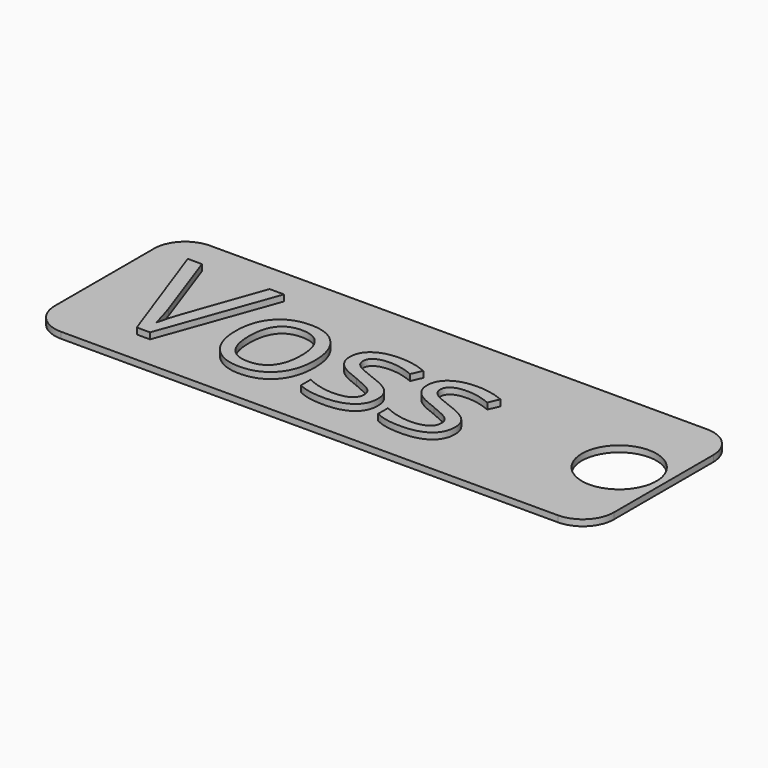
from build123d import *

# Parameters (mm, degrees)
F0_W         = 90
F0_H         = 30
F1_DEPTH     = 1
F2_R         = 5
F3_TEXT_SIZE = 26.041668995
F4_DEPTH     = 1
F6_D         = 12
F6_DEPTH     = 15.5
F6_TIP       = 3.6051637142


# Not quite as in the source:
# - Text() gives the source's letters only with a copy of the font that has no kerning and outlines rounded to 1/6400 em; it was checked with that copy


with BuildPart() as f1:
    # F0 (on Top) → F1 (new body)
    with BuildSketch(Plane.XY):
        Rectangle(F0_W, F0_H)
    extrude(amount=F1_DEPTH)

    # F2
    f2_edges = [f1.edges().sort_by_distance(p)[0] for p in [
        (-45, -15, 0.5),
        (45, -15, 0.5),
        (45, 15, 0.5),
        (-45, 15, 0.5),
    ]]
    fillet(f2_edges, radius=F2_R)

    # F3 (on face) → F4 (join)
    with BuildSketch(Plane.XY.offset(1)):
        with Locations((-38.750000298, -9.6428580582)):
            Text('Voss', F3_TEXT_SIZE, font='Open Sans', text_align=(TextAlign.LEFT, TextAlign.BOTTOM))
    extrude(amount=F4_DEPTH)

    # F6
    with Locations(Plane.XY.offset(1)):
        with Locations((37.8571413457, 0)):
            Hole(F6_D / 2, depth=F6_DEPTH)
            with Locations((0, 0, -(F6_DEPTH + F6_TIP / 2))):  # 118° drill point
                Cone(0, F6_D / 2, F6_TIP, mode=Mode.SUBTRACT)


solid = f1.part
